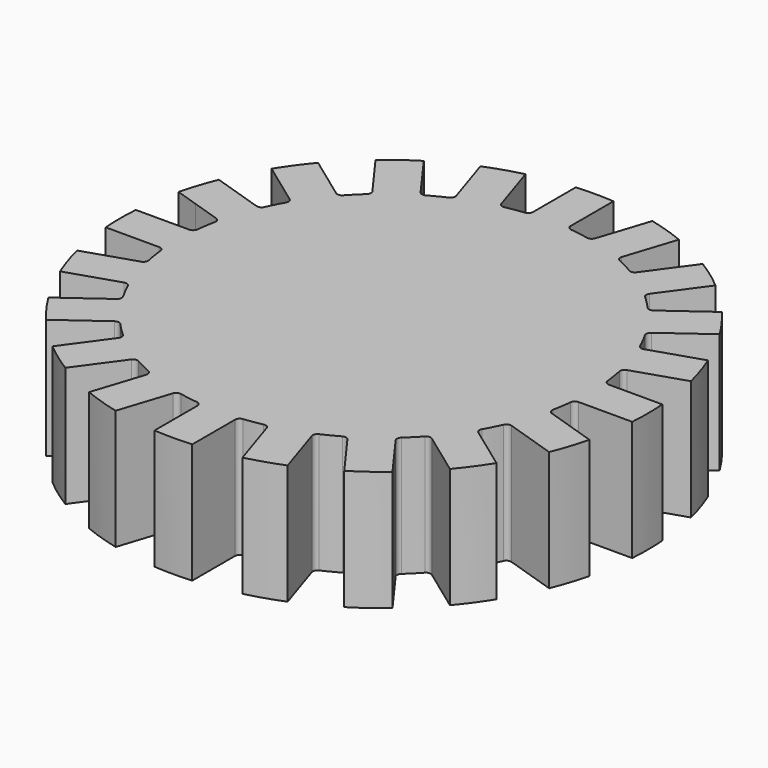
from build123d import *

# Parameters (mm, degrees)
F1_DEPTH = 5


# Not quite as in the source:
# - a feature names something its author has since deleted; it is built from what else it names


with BuildPart() as f1:
    # F0 (on Top) → F1 (new body)
    with BuildSketch(Plane.XY):
        with BuildLine():
            ThreePointArc((0.9630027506, 8.5459128069), (0, 8.6), (-0.9630027506, 8.5459128069))
            ThreePointArc((-0.9630027506, 8.5459128069), (-1.3453363993, 8.4941197291), (-1.7249622486, 8.4252302782))
            ThreePointArc((-1.7249622486, 8.4252302782), (-2.3394943883, 8.2756731453), (-2.9413732326, 8.0813565388))
            ThreePointArc((-2.9413732326, 8.0813565388), (-3.2514664019, 7.9616559984), (-3.5567023309, 7.8300618471))
            ThreePointArc((-3.5567023309, 7.8300618471), (-3.9043182978, 7.662656108), (-4.2440759244, 7.4798275079))
            ThreePointArc((-4.2440759244, 7.4798275079), (-5.0549531697, 6.9575461516), (-5.8022471061, 6.3477498785))
            ThreePointArc((-5.8022471061, 6.3477498785), (-6.0811183182, 6.0811183182), (-6.3477498785, 5.8022471061))
            ThreePointArc((-6.3477498785, 5.8022471061), (-6.9575461516, 5.0549531697), (-7.4798275079, 4.2440759244))
            ThreePointArc((-7.4798275079, 4.2440759244), (-7.662656108, 3.9043182978), (-7.8300618471, 3.5567023309))
            ThreePointArc((-7.8300618471, 3.5567023309), (-8.1790860401, 2.6575461516), (-8.4252302782, 1.7249622486))
            ThreePointArc((-8.4252302782, 1.7249622486), (-8.4941197291, 1.3453363993), (-8.5459128069, 0.9630027506))
            ThreePointArc((-8.5459128069, 0.9630027506), (-8.6, 0), (-8.5459128069, -0.9630027506))
            ThreePointArc((-8.5459128069, -0.9630027506), (-8.4941197291, -1.3453363993), (-8.4252302782, -1.7249622486))
            ThreePointArc((-8.4252302782, -1.7249622486), (-8.1790860401, -2.6575461516), (-7.8300618471, -3.5567023309))
            ThreePointArc((-7.8300618471, -3.5567023309), (-7.662656108, -3.9043182978), (-7.4798275079, -4.2440759244))
            ThreePointArc((-7.4798275079, -4.2440759244), (-6.9575461516, -5.0549531697), (-6.3477498785, -5.8022471061))
            ThreePointArc((-6.3477498785, -5.8022471061), (-6.0811183182, -6.0811183182), (-5.8022471061, -6.3477498785))
            ThreePointArc((-5.8022471061, -6.3477498785), (-5.0549531697, -6.9575461516), (-4.2440759244, -7.4798275079))
            ThreePointArc((-4.2440759244, -7.4798275079), (-3.9043182978, -7.662656108), (-3.5567023309, -7.8300618471))
            ThreePointArc((-3.5567023309, -7.8300618471), (-2.6575461516, -8.1790860401), (-1.7249622486, -8.4252302782))
            ThreePointArc((-1.7249622486, -8.4252302782), (-1.3453363993, -8.4941197291), (-0.9630027506, -8.5459128069))
            ThreePointArc((-0.9630027506, -8.5459128069), (0, -8.6), (0.9630027506, -8.5459128069))
            ThreePointArc((0.9630027506, -8.5459128069), (1.3453363993, -8.4941197291), (1.7249622486, -8.4252302782))
            ThreePointArc((1.7249622486, -8.4252302782), (2.6575461516, -8.1790860401), (3.5567023309, -7.8300618471))
            ThreePointArc((3.5567023309, -7.8300618471), (3.9043182978, -7.662656108), (4.2440759244, -7.4798275079))
            ThreePointArc((4.2440759244, -7.4798275079), (5.0549531697, -6.9575461516), (5.8022471061, -6.3477498785))
            ThreePointArc((5.8022471061, -6.3477498785), (6.0811183182, -6.0811183182), (6.3477498785, -5.8022471061))
            ThreePointArc((6.3477498785, -5.8022471061), (6.9575461516, -5.0549531697), (7.4798275079, -4.2440759244))
            ThreePointArc((7.4798275079, -4.2440759244), (7.662656108, -3.9043182978), (7.8300618471, -3.5567023309))
            ThreePointArc((7.8300618471, -3.5567023309), (8.1790860401, -2.6575461516), (8.4252302782, -1.7249622486))
            ThreePointArc((8.4252302782, -1.7249622486), (8.4941197291, -1.3453363993), (8.5459128069, -0.9630027506))
            ThreePointArc((8.5459128069, -0.9630027506), (8.6, 0), (8.5459128069, 0.9630027506))
            ThreePointArc((8.5459128069, 0.9630027506), (8.4941197291, 1.3453363993), (8.4252302782, 1.7249622486))
            ThreePointArc((8.4252302782, 1.7249622486), (8.1790860401, 2.6575461516), (7.8300618471, 3.5567023309))
            ThreePointArc((7.8300618471, 3.5567023309), (7.662656108, 3.9043182978), (7.4798275079, 4.2440759244))
            ThreePointArc((7.4798275079, 4.2440759244), (6.9575461516, 5.0549531697), (6.3477498785, 5.8022471061))
            ThreePointArc((6.3477498785, 5.8022471061), (6.0811183182, 6.0811183182), (5.8022471061, 6.3477498785))
            ThreePointArc((5.8022471061, 6.3477498785), (5.0549531697, 6.9575461516), (4.2440759244, 7.4798275079))
            ThreePointArc((4.2440759244, 7.4798275079), (3.9043182978, 7.662656108), (3.5567023309, 7.8300618471))
            ThreePointArc((3.5567023309, 7.8300618471), (3.2514664019, 7.9616559984), (2.9413732326, 8.0813565388))
            ThreePointArc((2.9413732326, 8.0813565388), (2.3394943883, 8.2756731453), (1.7249622486, 8.4252302782))
            ThreePointArc((1.7249622486, 8.4252302782), (1.3453363993, 8.4941197291), (0.9630027506, 8.5459128069))
        make_face()
        with BuildLine():
            ThreePointArc((-0.7853981634, 8.7446549652), (-0.8362688863, 8.6113865941), (-0.9630027506, 8.5459128069))
            ThreePointArc((-0.9630027506, 8.5459128069), (0, 8.6), (0.9630027506, 8.5459128069))
            ThreePointArc((0.9630027506, 8.5459128069), (0.8362688863, 8.6113865941), (0.7853981634, 8.7446549652))
            Line((0.7853981634, 8.7446549652), (0.7853981634, 10.9719255249))
            ThreePointArc((0.7853981634, 10.9719255249), (0, 11), (-0.7853981634, 10.9719255249))
            Line((-0.7853981634, 10.9719255249), (-0.7853981634, 8.7446549652))
        make_face()
        with BuildLine():
            ThreePointArc((-2.9413732326, 8.0813565388), (-2.3394943883, 8.2756731453), (-1.7249622486, 8.4252302782))
            ThreePointArc((-1.7249622486, 8.4252302782), (-1.865725829, 8.4483366324), (-1.955288953, 8.5593624672))
            Line((-1.955288953, 8.5593624672), (-2.643553407, 10.6776226466))
            ThreePointArc((-2.643553407, 10.6776226466), (-3.3991869381, 10.4616216792), (-4.1374694894, 10.192219887))
            Line((-4.1374694894, 10.192219887), (-3.4492050354, 8.0739597075))
            ThreePointArc((-3.4492050354, 8.0739597075), (-3.4564037764, 7.9314940369), (-3.5567023309, 7.8300618471))
            ThreePointArc((-3.5567023309, 7.8300618471), (-3.2514664019, 7.9616559984), (-2.9413732326, 8.0813565388))
        make_face()
        with BuildLine():
            ThreePointArc((1.955288953, 8.5593624672), (1.865725829, 8.4483366324), (1.7249622486, 8.4252302782))
            ThreePointArc((1.7249622486, 8.4252302782), (2.3394943883, 8.2756731453), (2.9413732326, 8.0813565388))
            ThreePointArc((2.9413732326, 8.0813565388), (3.2514664019, 7.9616559984), (3.5567023309, 7.8300618471))
            ThreePointArc((3.5567023309, 7.8300618471), (3.4564037764, 7.9314940369), (3.4492050354, 8.0739597075))
            Line((3.4492050354, 8.0739597075), (4.1374694894, 10.192219887))
            ThreePointArc((4.1374694894, 10.192219887), (3.3991869381, 10.4616216792), (2.643553407, 10.6776226466))
            Line((2.643553407, 10.6776226466), (1.955288953, 8.5593624672))
        make_face()
        with BuildLine():
            ThreePointArc((-5.8022471061, 6.3477498785), (-5.0549531697, 6.9575461516), (-4.2440759244, 7.4798275079))
            ThreePointArc((-4.2440759244, 7.4798275079), (-4.3850903009, 7.4583046181), (-4.5045787634, 7.5362199344))
            Line((-4.5045787634, 7.5362199344), (-5.8137355513, 9.3381196683))
            ThreePointArc((-5.8137355513, 9.3381196683), (-6.4656377752, 8.8991869381), (-7.0845364744, 8.4148287531))
            Line((-7.0845364744, 8.4148287531), (-6.4950961663, 7.6035337699))
            Line((-6.4950961663, 7.6035337699), (-5.7753796864, 6.6129290191))
            ThreePointArc((-5.7753796864, 6.6129290191), (-5.7382017827, 6.4752115814), (-5.8022471061, 6.3477498785))
        make_face()
        with BuildLine():
            ThreePointArc((4.5045787634, 7.5362199344), (4.3850903009, 7.4583046181), (4.2440759244, 7.4798275079))
            ThreePointArc((4.2440759244, 7.4798275079), (5.0549531697, 6.9575461516), (5.8022471061, 6.3477498785))
            ThreePointArc((5.8022471061, 6.3477498785), (5.7382017827, 6.4752115814), (5.7753796864, 6.6129290191))
            Line((5.7753796864, 6.6129290191), (7.0845364744, 8.4148287531))
            ThreePointArc((7.0845364744, 8.4148287531), (6.4656377752, 8.8991869381), (5.8137355513, 9.3381196683))
            Line((5.8137355513, 9.3381196683), (4.5045787634, 7.5362199344))
        make_face()
        with BuildLine():
            ThreePointArc((-7.4798275079, 4.2440759244), (-6.9575461516, 5.0549531697), (-6.3477498785, 5.8022471061))
            ThreePointArc((-6.3477498785, 5.8022471061), (-6.4752115814, 5.7382017827), (-6.6129290191, 5.7753796864))
            Line((-6.6129290191, 5.7753796864), (-8.4148287531, 7.0845364744))
            ThreePointArc((-8.4148287531, 7.0845364744), (-8.8991869381, 6.4656377752), (-9.3381196683, 5.8137355513))
            Line((-9.3381196683, 5.8137355513), (-7.5362199344, 4.5045787634))
            ThreePointArc((-7.5362199344, 4.5045787634), (-7.4583046181, 4.3850903009), (-7.4798275079, 4.2440759244))
        make_face()
        with BuildLine():
            ThreePointArc((6.6129290191, 5.7753796864), (6.4752115814, 5.7382017827), (6.3477498785, 5.8022471061))
            ThreePointArc((6.3477498785, 5.8022471061), (6.9575461516, 5.0549531697), (7.4798275079, 4.2440759244))
            ThreePointArc((7.4798275079, 4.2440759244), (7.4583046181, 4.3850903009), (7.5362199344, 4.5045787634))
            Line((7.5362199344, 4.5045787634), (9.3381196683, 5.8137355513))
            ThreePointArc((9.3381196683, 5.8137355513), (8.8991869381, 6.4656377752), (8.4148287531, 7.0845364744))
            Line((8.4148287531, 7.0845364744), (6.6129290191, 5.7753796864))
        make_face()
        with BuildLine():
            ThreePointArc((-8.4252302782, 1.7249622486), (-8.1790860401, 2.6575461516), (-7.8300618471, 3.5567023309))
            ThreePointArc((-7.8300618471, 3.5567023309), (-7.9314940369, 3.4564037764), (-8.0739597075, 3.4492050354))
            Line((-8.0739597075, 3.4492050354), (-10.192219887, 4.1374694894))
            ThreePointArc((-10.192219887, 4.1374694894), (-10.4616216792, 3.3991869381), (-10.6776226466, 2.643553407))
            Line((-10.6776226466, 2.643553407), (-9.7238881939, 2.3336662984))
            Line((-9.7238881939, 2.3336662984), (-8.5593624672, 1.955288953))
            ThreePointArc((-8.5593624672, 1.955288953), (-8.4483366324, 1.865725829), (-8.4252302782, 1.7249622486))
        make_face()
        with BuildLine():
            ThreePointArc((8.0739597075, 3.4492050354), (7.9314940369, 3.4564037764), (7.8300618471, 3.5567023309))
            ThreePointArc((7.8300618471, 3.5567023309), (8.1790860401, 2.6575461516), (8.4252302782, 1.7249622486))
            ThreePointArc((8.4252302782, 1.7249622486), (8.4483366324, 1.865725829), (8.5593624672, 1.955288953))
            Line((8.5593624672, 1.955288953), (10.6776226466, 2.643553407))
            ThreePointArc((10.6776226466, 2.643553407), (10.4616216792, 3.3991869381), (10.192219887, 4.1374694894))
            Line((10.192219887, 4.1374694894), (8.0739597075, 3.4492050354))
        make_face()
        with BuildLine():
            ThreePointArc((-8.5459128069, -0.9630027506), (-8.6, 0), (-8.5459128069, 0.9630027506))
            ThreePointArc((-8.5459128069, 0.9630027506), (-8.6113865941, 0.8362688863), (-8.7446549652, 0.7853981634))
            Line((-8.7446549652, 0.7853981634), (-10.9719255249, 0.7853981634))
            ThreePointArc((-10.9719255249, 0.7853981634), (-11, 0), (-10.9719255249, -0.7853981634))
            Line((-10.9719255249, -0.7853981634), (-8.7446549652, -0.7853981634))
            ThreePointArc((-8.7446549652, -0.7853981634), (-8.6113865941, -0.8362688863), (-8.5459128069, -0.9630027506))
        make_face()
        with BuildLine():
            ThreePointArc((8.7446549652, 0.7853981634), (8.6113865941, 0.8362688863), (8.5459128069, 0.9630027506))
            ThreePointArc((8.5459128069, 0.9630027506), (8.6, 0), (8.5459128069, -0.9630027506))
            ThreePointArc((8.5459128069, -0.9630027506), (8.6113865941, -0.8362688863), (8.7446549652, -0.7853981634))
            Line((8.7446549652, -0.7853981634), (10.9719255249, -0.7853981634))
            ThreePointArc((10.9719255249, -0.7853981634), (11, 0), (10.9719255249, 0.7853981634))
            Line((10.9719255249, 0.7853981634), (8.7446549652, 0.7853981634))
        make_face()
        with BuildLine():
            ThreePointArc((-7.8300618471, -3.5567023309), (-8.1790860401, -2.6575461516), (-8.4252302782, -1.7249622486))
            ThreePointArc((-8.4252302782, -1.7249622486), (-8.4483366324, -1.865725829), (-8.5593624672, -1.955288953))
            Line((-8.5593624672, -1.955288953), (-10.6776226466, -2.643553407))
            ThreePointArc((-10.6776226466, -2.643553407), (-10.4616216792, -3.3991869381), (-10.192219887, -4.1374694894))
            Line((-10.192219887, -4.1374694894), (-8.0739597075, -3.4492050354))
            ThreePointArc((-8.0739597075, -3.4492050354), (-7.9314940369, -3.4564037764), (-7.8300618471, -3.5567023309))
        make_face()
        with BuildLine():
            ThreePointArc((8.5593624672, -1.955288953), (8.4483366324, -1.865725829), (8.4252302782, -1.7249622486))
            ThreePointArc((8.4252302782, -1.7249622486), (8.1790860401, -2.6575461516), (7.8300618471, -3.5567023309))
            ThreePointArc((7.8300618471, -3.5567023309), (7.9314940369, -3.4564037764), (8.0739597075, -3.4492050354))
            Line((8.0739597075, -3.4492050354), (10.192219887, -4.1374694894))
            ThreePointArc((10.192219887, -4.1374694894), (10.4616216792, -3.3991869381), (10.6776226466, -2.643553407))
            Line((10.6776226466, -2.643553407), (8.5593624672, -1.955288953))
        make_face()
        with BuildLine():
            ThreePointArc((-6.3477498785, -5.8022471061), (-6.9575461516, -5.0549531697), (-7.4798275079, -4.2440759244))
            ThreePointArc((-7.4798275079, -4.2440759244), (-7.4583046181, -4.3850903009), (-7.5362199344, -4.5045787634))
            Line((-7.5362199344, -4.5045787634), (-9.3381196683, -5.8137355513))
            ThreePointArc((-9.3381196683, -5.8137355513), (-8.8991869381, -6.4656377752), (-8.4148287531, -7.0845364744))
            Line((-8.4148287531, -7.0845364744), (-6.6129290191, -5.7753796864))
            ThreePointArc((-6.6129290191, -5.7753796864), (-6.4752115814, -5.7382017827), (-6.3477498785, -5.8022471061))
        make_face()
        with BuildLine():
            ThreePointArc((7.5362199344, -4.5045787634), (7.4583046181, -4.3850903009), (7.4798275079, -4.2440759244))
            ThreePointArc((7.4798275079, -4.2440759244), (6.9575461516, -5.0549531697), (6.3477498785, -5.8022471061))
            ThreePointArc((6.3477498785, -5.8022471061), (6.4752115814, -5.7382017827), (6.6129290191, -5.7753796864))
            Line((6.6129290191, -5.7753796864), (8.4148287531, -7.0845364744))
            ThreePointArc((8.4148287531, -7.0845364744), (8.8991869381, -6.4656377752), (9.3381196683, -5.8137355513))
            Line((9.3381196683, -5.8137355513), (7.5362199344, -4.5045787634))
        make_face()
        with BuildLine():
            ThreePointArc((-4.2440759244, -7.4798275079), (-5.0549531697, -6.9575461516), (-5.8022471061, -6.3477498785))
            ThreePointArc((-5.8022471061, -6.3477498785), (-5.7382017827, -6.4752115814), (-5.7753796864, -6.6129290191))
            Line((-5.7753796864, -6.6129290191), (-7.0845364744, -8.4148287531))
            ThreePointArc((-7.0845364744, -8.4148287531), (-6.4656377752, -8.8991869381), (-5.8137355513, -9.3381196683))
            Line((-5.8137355513, -9.3381196683), (-4.5045787634, -7.5362199344))
            ThreePointArc((-4.5045787634, -7.5362199344), (-4.3850903009, -7.4583046181), (-4.2440759244, -7.4798275079))
        make_face()
        with BuildLine():
            ThreePointArc((5.7753796864, -6.6129290191), (5.7382017827, -6.4752115814), (5.8022471061, -6.3477498785))
            ThreePointArc((5.8022471061, -6.3477498785), (5.0549531697, -6.9575461516), (4.2440759244, -7.4798275079))
            ThreePointArc((4.2440759244, -7.4798275079), (4.3850903009, -7.4583046181), (4.5045787634, -7.5362199344))
            Line((4.5045787634, -7.5362199344), (5.8137355513, -9.3381196683))
            ThreePointArc((5.8137355513, -9.3381196683), (6.4656377752, -8.8991869381), (7.0845364744, -8.4148287531))
            Line((7.0845364744, -8.4148287531), (5.7753796864, -6.6129290191))
        make_face()
        with BuildLine():
            ThreePointArc((-1.7249622486, -8.4252302782), (-2.6575461516, -8.1790860401), (-3.5567023309, -7.8300618471))
            ThreePointArc((-3.5567023309, -7.8300618471), (-3.4564037764, -7.9314940369), (-3.4492050354, -8.0739597075))
            Line((-3.4492050354, -8.0739597075), (-4.1374694894, -10.192219887))
            ThreePointArc((-4.1374694894, -10.192219887), (-3.3991869381, -10.4616216792), (-2.643553407, -10.6776226466))
            Line((-2.643553407, -10.6776226466), (-1.955288953, -8.5593624672))
            ThreePointArc((-1.955288953, -8.5593624672), (-1.865725829, -8.4483366324), (-1.7249622486, -8.4252302782))
        make_face()
        with BuildLine():
            ThreePointArc((3.4492050354, -8.0739597075), (3.4564037764, -7.9314940369), (3.5567023309, -7.8300618471))
            ThreePointArc((3.5567023309, -7.8300618471), (2.6575461516, -8.1790860401), (1.7249622486, -8.4252302782))
            ThreePointArc((1.7249622486, -8.4252302782), (1.865725829, -8.4483366324), (1.955288953, -8.5593624672))
            Line((1.955288953, -8.5593624672), (2.643553407, -10.6776226466))
            ThreePointArc((2.643553407, -10.6776226466), (3.3991869381, -10.4616216792), (4.1374694894, -10.192219887))
            Line((4.1374694894, -10.192219887), (3.4492050354, -8.0739597075))
        make_face()
        with BuildLine():
            ThreePointArc((0.9630027506, -8.5459128069), (0, -8.6), (-0.9630027506, -8.5459128069))
            ThreePointArc((-0.9630027506, -8.5459128069), (-0.8362688863, -8.6113865941), (-0.7853981634, -8.7446549652))
            Line((-0.7853981634, -8.7446549652), (-0.7853981634, -10.9719255249))
            ThreePointArc((-0.7853981634, -10.9719255249), (0, -11), (0.7853981634, -10.9719255249))
            Line((0.7853981634, -10.9719255249), (0.7853981634, -8.7446549652))
            ThreePointArc((0.7853981634, -8.7446549652), (0.8362688863, -8.6113865941), (0.9630027506, -8.5459128069))
        make_face()
    extrude(amount=F1_DEPTH)


solid = f1.part
